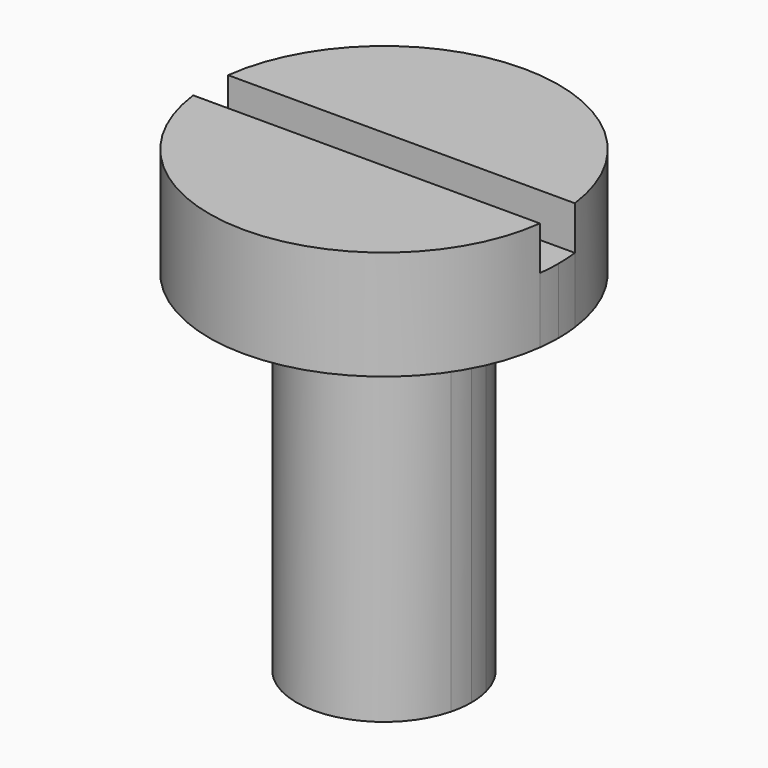
from build123d import *

# Parameters (mm, degrees)
F1_DEPTH = 8
F2_DEPTH = 2.5
F3_DEPTH = 1.5


# Not quite as in the source:
# - a feature names something its author has since deleted; it is built from what else it names


with BuildPart() as f1:
    # F0 (on Top) → F1 (new body)
    with BuildSketch(Plane.XY):
        with BuildLine():
            Line((-1.9364916731, 0.5), (1.9364916731, 0.5))
            ThreePointArc((1.9364916731, 0.5), (0, 2), (-1.9364916731, 0.5))
        make_face()
        with BuildLine():
            ThreePointArc((2, 0), (1.9840593925, 0.252008585), (1.9364916731, 0.5))
            Line((1.9364916731, 0.5), (-1.9364916731, 0.5))
            ThreePointArc((-1.9364916731, 0.5), (-2, 0), (-1.9364916731, -0.5))
            Line((-1.9364916731, -0.5), (1.9364916731, -0.5))
            ThreePointArc((1.9364916731, -0.5), (1.9840593925, -0.252008585), (2, 0))
        make_face()
        with BuildLine():
            ThreePointArc((-1.9364916731, -0.5), (0, -2), (1.9364916731, -0.5))
            Line((1.9364916731, -0.5), (-1.9364916731, -0.5))
        make_face()
    extrude(amount=-F1_DEPTH)

    # F0 (on Top) → F2 (join)
    with BuildSketch(Plane.XY):
        with BuildLine():
            ThreePointArc((-3.9686269666, -0.5), (0, -4), (3.9686269666, -0.5))
            Line((3.9686269666, -0.5), (1.9364916731, -0.5))
            ThreePointArc((1.9364916731, -0.5), (0, -2), (-1.9364916731, -0.5))
            Line((-1.9364916731, -0.5), (-3.9686269666, -0.5))
        make_face()
        with BuildLine():
            Line((1.9364916731, 0.5), (3.9686269666, 0.5))
            ThreePointArc((3.9686269666, 0.5), (0, 4), (-3.9686269666, 0.5))
            Line((-3.9686269666, 0.5), (-1.9364916731, 0.5))
            ThreePointArc((-1.9364916731, 0.5), (0, 2), (1.9364916731, 0.5))
        make_face()
        with BuildLine():
            Line((-1.9364916731, 0.5), (1.9364916731, 0.5))
            ThreePointArc((1.9364916731, 0.5), (0, 2), (-1.9364916731, 0.5))
        make_face()
        with BuildLine():
            ThreePointArc((-1.9364916731, -0.5), (0, -2), (1.9364916731, -0.5))
            Line((1.9364916731, -0.5), (-1.9364916731, -0.5))
        make_face()
    extrude(amount=F2_DEPTH)

    # F0 (on Top) → F3 (join)
    with BuildSketch(Plane.XY):
        with BuildLine():
            Line((-1.9364916731, 0.5), (-3.9686269666, 0.5))
            ThreePointArc((-3.9686269666, 0.5), (-4, 0), (-3.9686269666, -0.5))
            Line((-3.9686269666, -0.5), (-1.9364916731, -0.5))
            ThreePointArc((-1.9364916731, -0.5), (-2, 0), (-1.9364916731, 0.5))
        make_face()
        with BuildLine():
            ThreePointArc((2, 0), (1.9840593925, 0.252008585), (1.9364916731, 0.5))
            Line((1.9364916731, 0.5), (-1.9364916731, 0.5))
            ThreePointArc((-1.9364916731, 0.5), (-2, 0), (-1.9364916731, -0.5))
            Line((-1.9364916731, -0.5), (1.9364916731, -0.5))
            ThreePointArc((1.9364916731, -0.5), (1.9840593925, -0.252008585), (2, 0))
        make_face()
        with BuildLine():
            ThreePointArc((3.9686269666, -0.5), (3.9921490369, -0.2504916502), (4, 0))
            ThreePointArc((4, 0), (3.9921490369, 0.2504916502), (3.9686269666, 0.5))
            Line((3.9686269666, 0.5), (1.9364916731, 0.5))
            ThreePointArc((1.9364916731, 0.5), (1.9840593925, 0.252008585), (2, 0))
            ThreePointArc((2, 0), (1.9840593925, -0.252008585), (1.9364916731, -0.5))
            Line((1.9364916731, -0.5), (3.9686269666, -0.5))
        make_face()
    extrude(amount=F3_DEPTH)


solid = f1.part
